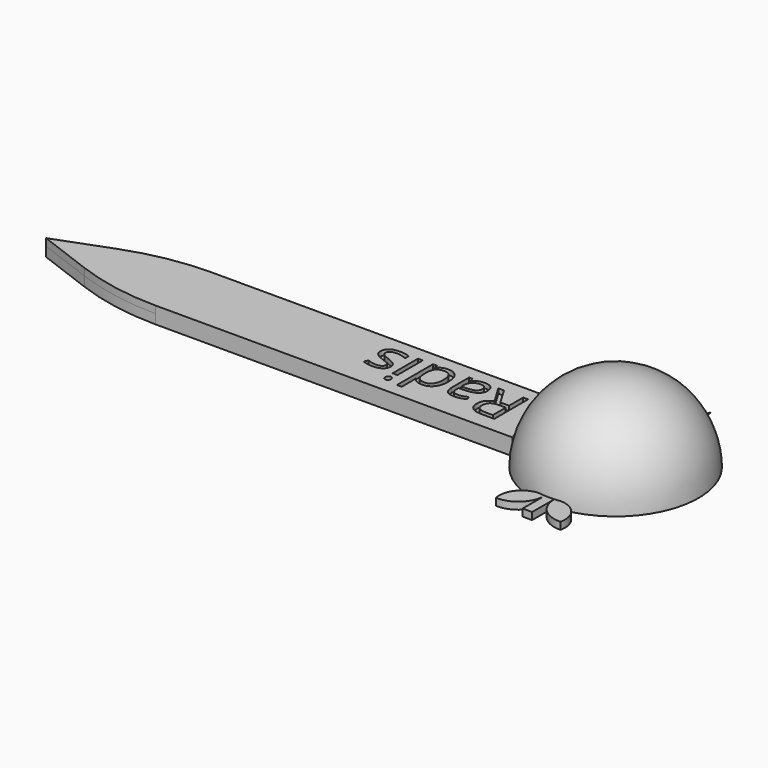
from build123d import *

# Parameters (mm, degrees)
F0_W         = 100
F0_H         = 15
F1_DEPTH     = 2
F2_R         = 50
F4_ANGLE     = 180
F6_DEPTH     = 1.5
F7_TEXT_SIZE = 12.5060569391
F8_DEPTH     = 1


# Not quite as in the source:
# - Text() gives the source's letters only with a copy of the font that has no kerning and outlines rounded to 1/6400 em; it was checked with that copy


with BuildPart() as f1:
    # F0 (on Top) → F1 (new body)
    with BuildSketch(Plane.XY):
        with Locations((70, 0)):
            Rectangle(F0_W, F0_H)
        Polygon((20, -7.5), (20, 7.5), (0, 0), align=None)
    extrude(amount=F1_DEPTH)

    # F2
    f2_edges = [f1.edges().sort_by_distance(p)[0] for p in [
        (20, -7.5, 1),
        (20, 7.5, 1),
    ]]
    fillet(f2_edges, radius=F2_R)

    # F3 (on face) → F4 (revolve)
    with BuildSketch(Plane(origin=(0, 0, 0), x_dir=(1, 0, 0), z_dir=(0, 0, -1))):
        with BuildLine():
            Line((120, -17.5), (120, 17.5))
            ThreePointArc((120, 17.5), (102.8691395237, 3.5754187646), (113, -16.0390149323))
            ThreePointArc((113, -16.0390149323), (116.4245812354, -17.1308604763), (120, -17.5))
        make_face()
        with BuildLine():
            ThreePointArc((120, -17.5), (116.4245812354, -17.1308604763), (113, -16.0390149323))
            ThreePointArc((113, -16.0390149323), (117.634826678, -19.6330215848), (120, -25))
            Line((120, -25), (120, -17.5))
        make_face()
    revolve(axis=Axis((120, 0, 0), (0, 1, 0)), revolution_arc=F4_ANGLE)

    # F5 (on face) + F1_face1 (on face) → F6 (join)
    with BuildSketch(Plane(origin=(0, 0, 0), x_dir=(1, 0, 0), z_dir=(0, 0, -1))):
        with BuildLine():
            Line((121.0126270091, 23.2601012398), (120.0126316838, 23.2570435844))
            Line((120.0126316838, 23.2570435844), (119.0126363584, 23.253985929))
            Line((119.0126363584, 23.253985929), (119.0303123559, 17.4731138001))
            ThreePointArc((119.0303123559, 17.4731138001), (117.2914360229, 21.4904868971), (113.1814420223, 22.9974463582))
            ThreePointArc((113.1814420223, 22.9974463582), (113.9842351085, 19.2333232973), (117.3073070101, 17.2915992454))
            Line((117.3073070101, 17.2915992454), (122.7543861476, 17.3082546141))
            ThreePointArc((122.7543861476, 17.3082546141), (126.0655217221, 19.2702638812), (126.8452811224, 23.0392258649))
            ThreePointArc((126.8452811224, 23.0392258649), (122.7445794551, 21.5071608085), (121.0303030066, 17.4792291109))
            Line((121.0303030066, 17.4792291109), (121.0126270091, 23.2601012398))
        make_face()
    with BuildSketch(Plane(origin=(56.662373143, 0, 2), x_dir=(1, 0, 0), z_dir=(0, 0, 1))):
        with BuildLine():
            ThreePointArc((47.6532397157, -7.5), (45.9522882063, 0), (47.6532397157, 7.5))
            Line((47.6532397157, 7.5), (-27.5956440543, 7.5))
            ThreePointArc((-27.5956440543, 7.5), (-36.516884329, 6.6976775058), (-45.1518161338, 4.3164588785))
            Line((-45.1518161338, 4.3164588785), (-56.662373143, 0))
            Line((-56.662373143, 0), (-45.1518161338, -4.3164588785))
            ThreePointArc((-45.1518161338, -4.3164588785), (-36.516884329, -6.6976775058), (-27.5956440543, -7.5))
            Line((-27.5956440543, -7.5), (47.6532397157, -7.5))
        make_face()
    extrude(amount=-F6_DEPTH, dir=(0, 0, -1))

    # F7 (on face) → F8 (cut)
    with BuildSketch(Plane.XY.offset(3.5)):
        with Locations(Location((99.0443388, 4.7005452216), (0, 0, 180))):
            Text('Radis', F7_TEXT_SIZE, font='Open Sans', text_align=(TextAlign.LEFT, TextAlign.BOTTOM))
    extrude(amount=-F8_DEPTH, mode=Mode.SUBTRACT)


solid = f1.part
